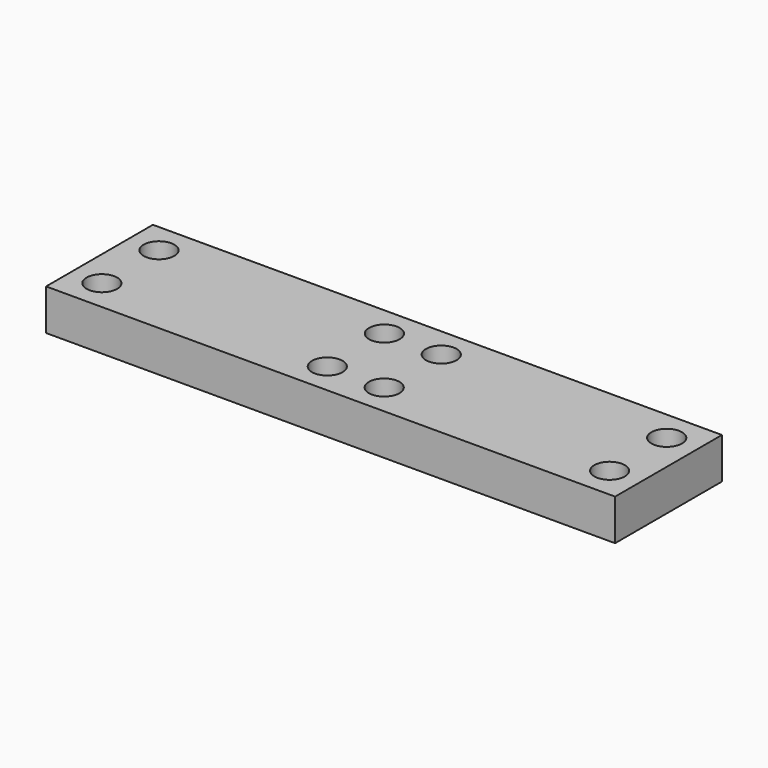
from build123d import *

# Parameters (mm, degrees)
F1_DEPTH = 4.7625


# Not quite as in the source:
# - a length typed as a fraction of an inch, garbled in the dataset ("3 / 203.2 mm" for 3/8 in), is restored


with BuildPart() as f1:
    # F0 (on Top) → F1 (new body)
    with BuildSketch(Plane.XY):
        with BuildLine():
            Line((-3.302, 5.9590800321), (-3.302, 7.747))
            Line((-3.302, 7.747), (-29.464, 7.747))
            Line((-29.464, 7.747), (-29.464, 5.9590800321))
            ThreePointArc((-29.464, 5.9590800321), (-28.2067641431, 5.4383158891), (-27.686, 4.1810800321))
            ThreePointArc((-27.686, 4.1810800321), (-28.2067641431, 2.9238441752), (-29.464, 2.4030800321))
            Line((-29.464, 2.4030800321), (-29.464, -2.3199413316))
            ThreePointArc((-29.464, -2.3199413316), (-28.2067641431, -2.8407054746), (-27.686, -4.0979413316))
            ThreePointArc((-27.686, -4.0979413316), (-28.2067641431, -5.3551771885), (-29.464, -5.8759413316))
            Line((-29.464, -5.8759413316), (-29.464, -7.747))
            Line((-29.464, -7.747), (-3.302, -7.747))
            Line((-3.302, -7.747), (-3.302, -5.8759413316))
            ThreePointArc((-3.302, -5.8759413316), (-5.08, -4.0979413316), (-3.302, -2.3199413316))
            Line((-3.302, -2.3199413316), (-3.302, 2.4030800321))
            ThreePointArc((-3.302, 2.4030800321), (-5.08, 4.1810800321), (-3.302, 5.9590800321))
        make_face()
        with BuildLine():
            Line((-29.464, 5.9590800321), (-29.464, 7.747))
            Line((-29.464, 7.747), (-33.02, 7.747))
            Line((-33.02, 7.747), (-33.02, -7.747))
            Line((-33.02, -7.747), (-29.464, -7.747))
            Line((-29.464, -7.747), (-29.464, -5.8759413316))
            ThreePointArc((-29.464, -5.8759413316), (-31.242, -4.0979413316), (-29.464, -2.3199413316))
            Line((-29.464, -2.3199413316), (-29.464, 2.4030800321))
            ThreePointArc((-29.464, 2.4030800321), (-31.242, 4.1810800321), (-29.464, 5.9590800321))
        make_face()
        with BuildLine():
            Line((29.464, 5.9590800321), (29.464, 7.747))
            Line((29.464, 7.747), (3.302, 7.747))
            Line((3.302, 7.747), (3.302, 5.9590800321))
            ThreePointArc((3.302, 5.9590800321), (4.5592358569, 5.4383158891), (5.08, 4.1810800321))
            ThreePointArc((5.08, 4.1810800321), (4.5592358569, 2.9238441752), (3.302, 2.4030800321))
            Line((3.302, 2.4030800321), (3.302, -2.3199413316))
            ThreePointArc((3.302, -2.3199413316), (4.5592358569, -2.8407054746), (5.08, -4.0979413316))
            ThreePointArc((5.08, -4.0979413316), (4.5592358569, -5.3551771885), (3.302, -5.8759413316))
            Line((3.302, -5.8759413316), (3.302, -7.747))
            Line((3.302, -7.747), (29.464, -7.747))
            Line((29.464, -7.747), (29.464, -5.8759413316))
            ThreePointArc((29.464, -5.8759413316), (27.686, -4.0979413316), (29.464, -2.3199413316))
            Line((29.464, -2.3199413316), (29.464, 2.4030800321))
            ThreePointArc((29.464, 2.4030800321), (27.686, 4.1810800321), (29.464, 5.9590800321))
        make_face()
        with BuildLine():
            Line((33.02, -7.747), (33.02, 7.747))
            Line((33.02, 7.747), (29.464, 7.747))
            Line((29.464, 7.747), (29.464, 5.9590800321))
            ThreePointArc((29.464, 5.9590800321), (30.7212358569, 5.4383158891), (31.242, 4.1810800321))
            ThreePointArc((31.242, 4.1810800321), (30.7212358569, 2.9238441752), (29.464, 2.4030800321))
            Line((29.464, 2.4030800321), (29.464, -2.3199413316))
            ThreePointArc((29.464, -2.3199413316), (30.7212358569, -2.8407054746), (31.242, -4.0979413316))
            ThreePointArc((31.242, -4.0979413316), (30.7212358569, -5.3551771885), (29.464, -5.8759413316))
            Line((29.464, -5.8759413316), (29.464, -7.747))
            Line((29.464, -7.747), (33.02, -7.747))
        make_face()
        with BuildLine():
            Line((3.302, 5.9590800321), (3.302, 7.747))
            Line((3.302, 7.747), (-3.302, 7.747))
            Line((-3.302, 7.747), (-3.302, 5.9590800321))
            ThreePointArc((-3.302, 5.9590800321), (-2.0447641431, 5.4383158891), (-1.524, 4.1810800321))
            ThreePointArc((-1.524, 4.1810800321), (-2.0447641431, 2.9238441752), (-3.302, 2.4030800321))
            Line((-3.302, 2.4030800321), (-3.302, -2.3199413316))
            ThreePointArc((-3.302, -2.3199413316), (-2.0447641431, -2.8407054746), (-1.524, -4.0979413316))
            ThreePointArc((-1.524, -4.0979413316), (-2.0447641431, -5.3551771885), (-3.302, -5.8759413316))
            Line((-3.302, -5.8759413316), (-3.302, -7.747))
            Line((-3.302, -7.747), (3.302, -7.747))
            Line((3.302, -7.747), (3.302, -5.8759413316))
            ThreePointArc((3.302, -5.8759413316), (1.524, -4.0979413316), (3.302, -2.3199413316))
            Line((3.302, -2.3199413316), (3.302, 2.4030800321))
            ThreePointArc((3.302, 2.4030800321), (1.524, 4.1810800321), (3.302, 5.9590800321))
        make_face()
    extrude(amount=F1_DEPTH)


solid = f1.part
